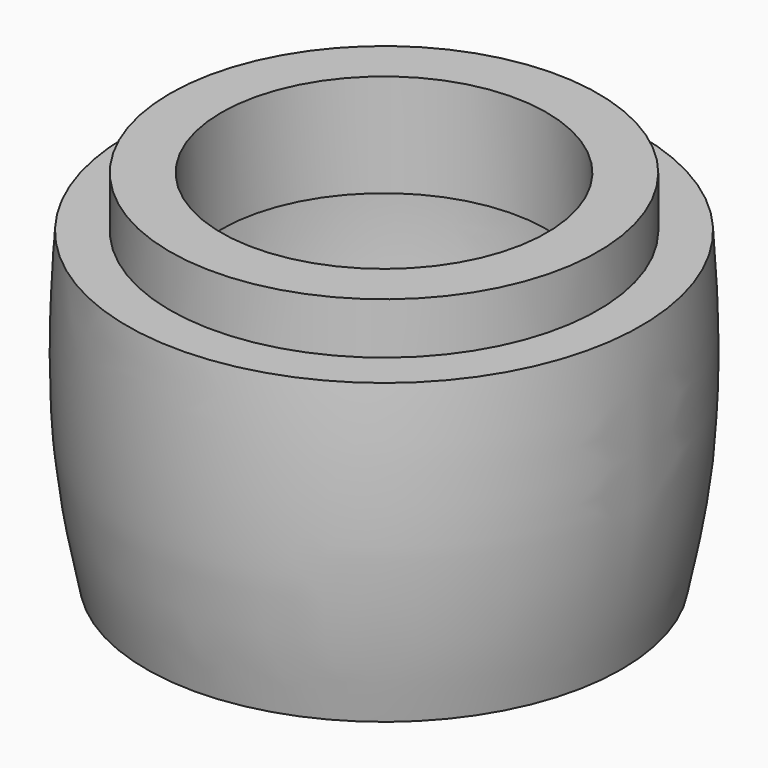
from build123d import *

# Parameters (mm, degrees)
F3_T = -3


# Not quite as in the source:
# - a feature of the source that left no trace in its solid (it failed there, or was rolled back) is left out


with BuildPart() as f2:
    # F1 (on face) → F2 (revolve)
    with BuildSketch(Plane.XZ):
        with BuildLine():
            Line((-12.5, -5), (-15, -5))
            add(Edge.make_bspline(
                [(-15, -5), (-15.2242291382, -7.9082660222), (-15.4829896575, -15.4302819777), (-14.3790599241, -20.605744182), (-13.8805727597, -23)],
                knots=[0.0395283873, 0.0395283873, 0.0395283873, 0.0395283873, 0.5201151217, 0.8906255687, 0.8906255687, 0.8906255687, 0.8906255687], degree=3))
            Line((-13.8805727597, -23), (0, -23))
            Line((0, -23), (0, -2))
            Line((0, -2), (-12.5, -2))
            Line((-12.5, -2), (-12.5, -5))
        make_face()
    revolve(axis=Axis((0, 0, -13.5), (0, 0, -1)))

    # F3
    f3_openings = [f2.faces().sort_by_distance(p)[0] for p in [
        (0, 0, -2),
    ]]
    offset(amount=F3_T, openings=f3_openings, kind=Kind.INTERSECTION)


solid = f2.part
